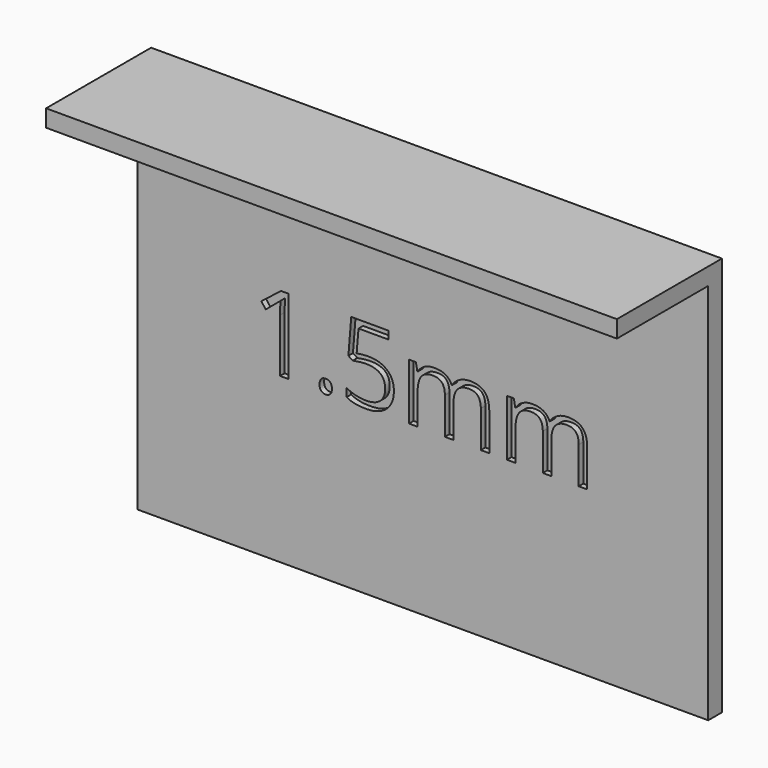
from build123d import *

# Parameters (mm, degrees)
F0_W         = 50
F0_H         = 35
F1_DEPTH     = 1.5
F2_W         = 50
F2_H         = 1.5
F3_DEPTH     = 10
F4_TEXT_SIZE = 9.2205734044
F5_DEPTH     = 0.5


# Not quite as in the source:
# - Text() gives the source's letters only with a copy of the font that has no kerning and outlines rounded to 1/6400 em; it was checked with that copy


with BuildPart() as f1:
    # F0 (on Front) → F1 (new body)
    with BuildSketch(Plane.XZ):
        Rectangle(F0_W, F0_H)
    extrude(amount=F1_DEPTH)

    # F2 (on face) → F3 (join)
    with BuildSketch(Plane.XZ.offset(1.5)):
        with Locations((0, 16.75)):
            Rectangle(F2_W, F2_H)
    extrude(amount=F3_DEPTH)

    # F4 (on face) → F5 (cut)
    with BuildSketch(Plane.XZ.offset(1.5)):
        with Locations((-15, -3.1405159953)):
            Text('1.5mm', F4_TEXT_SIZE, font='Open Sans', text_align=(TextAlign.LEFT, TextAlign.BOTTOM))
    extrude(amount=-F5_DEPTH, mode=Mode.SUBTRACT)


solid = f1.part
